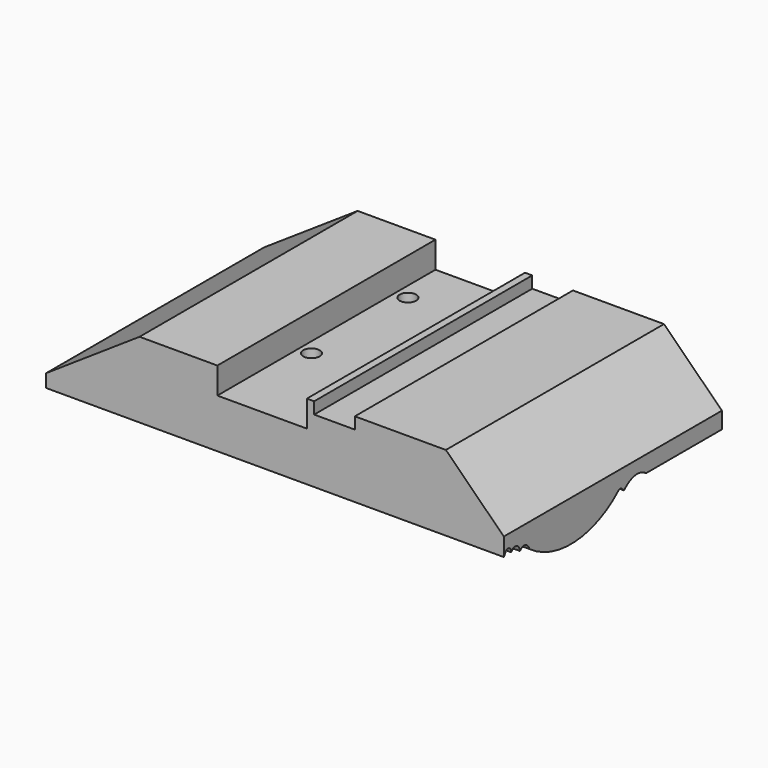
from build123d import *

# Parameters (mm, degrees)
F1_DEPTH      = 68.072
F1_DEPTH_BACK = 68.072
F2_R          = 4.1275
F3_DEPTH      = 13.97
F5_DEPTH      = 228.6
F6_DEPTH      = 228.6


# Not quite as in the source:
# - a feature names something its author has since deleted; it is built from what else it names


with BuildPart() as f1:
    # F0 (on Front) → F1 (new body, two sides)
    with BuildSketch(Plane.XZ) as f1_sk:
        Polygon((-114.3, 0), (0, 0), (114.3, 0), (114.3, 20.32), (85.358465722, 48.9655555556), (39.892465722, 48.9655555556), (39.892465722, 43.1235555556), (19.572465722, 43.1235555556), (19.572465722, 48.9655555556), (15.940265722, 48.9655555556), (15.940265722, 35.7575555556), (-28.763734278, 35.7575555556), (-28.763734278, 48.9655555556), (-67.625734278, 48.9655555556), (-114.3, 17.78), align=None)
    extrude(amount=F1_DEPTH)
    extrude(f1_sk.sketch, amount=-F1_DEPTH_BACK)

    # F2 (on face) → F3 (cut)
    with BuildSketch(Plane.XY.offset(35.7575555556)):
        with Locations((-22.413734278, 42.926)):
            Circle(F2_R)
        with Locations((9.590265722, 42.926)):
            Circle(F2_R)
        with Locations((9.590265722, -17.272)):
            Circle(F2_R)
        with Locations((-22.413734278, -17.272)):
            Circle(F2_R)
    extrude(amount=-F3_DEPTH, mode=Mode.SUBTRACT)

    # F4 (on face) → F5 (cut)
    with BuildSketch(Plane.YZ.offset(114.3)):
        with BuildLine():
            ThreePointArc((-28.7846772927, 0), (-41.092836195, 2.5095205348), (-52.197, 8.382))
            ThreePointArc((-52.197, 8.382), (-53.0628215245, 10.1004124317), (-54.6900965273, 11.1273322254))
            ThreePointArc((-54.6900965273, 11.1273322254), (-55.6077664174, 11.233907182), (-56.5009973943, 10.9980795532))
            ThreePointArc((-56.5009973943, 10.9980795532), (-57.2399299218, 10.5397598563), (-57.8612, 9.9314))
            ThreePointArc((-57.8612, 9.9314), (-58.0475109479, 9.8713617946), (-58.1624396145, 10.0298160687))
            Line((-58.1624396145, 10.0298160687), (-58.2733862102, 10.82482934))
            ThreePointArc((-58.2733862102, 10.82482934), (-60.2066850368, 13.0247678359), (-62.9914626479, 12.1179120615))
            Line((-62.9914626479, 12.1179120615), (-63.4766221046, 11.5155344829))
            Line((-63.4766221046, 11.5155344829), (-63.6741071939, 12.5305661932))
            ThreePointArc((-63.6741071939, 12.5305661932), (-65.141327886, 13.96093331), (-66.995896399, 13.0895767361))
            Line((-66.995896399, 13.0895767361), (-68.072, 11.2702753395))
            Line((-68.072, 11.2702753395), (-68.072, 0))
            Line((-68.072, 0), (-28.7846772927, 0))
        make_face()
    extrude(amount=-F5_DEPTH, mode=Mode.SUBTRACT)

    # F4 (on face) → F6 (cut)
    with BuildSketch(Plane.YZ.offset(114.3)):
        with BuildLine():
            ThreePointArc((3.5306, 11.43), (-9.0647706891, 3.3847479258), (-23.622, 0))
            Line((-23.622, 0), (68.072, 0))
            Line((68.072, 0), (68.072, 12.065))
            Line((68.072, 12.065), (20.6756, 12.065))
            ThreePointArc((20.6756, 12.065), (16.8687140076, 13.8395100393), (12.6746, 13.6144))
            ThreePointArc((12.6746, 13.6144), (9.5960531105, 12.2103950232), (6.985, 10.0584))
            Line((6.985, 10.0584), (5.6642, 11.43))
            ThreePointArc((5.6642, 11.43), (4.5974, 11.8463817681), (3.5306, 11.43))
        make_face()
    extrude(amount=-F6_DEPTH, mode=Mode.SUBTRACT)


solid = f1.part
